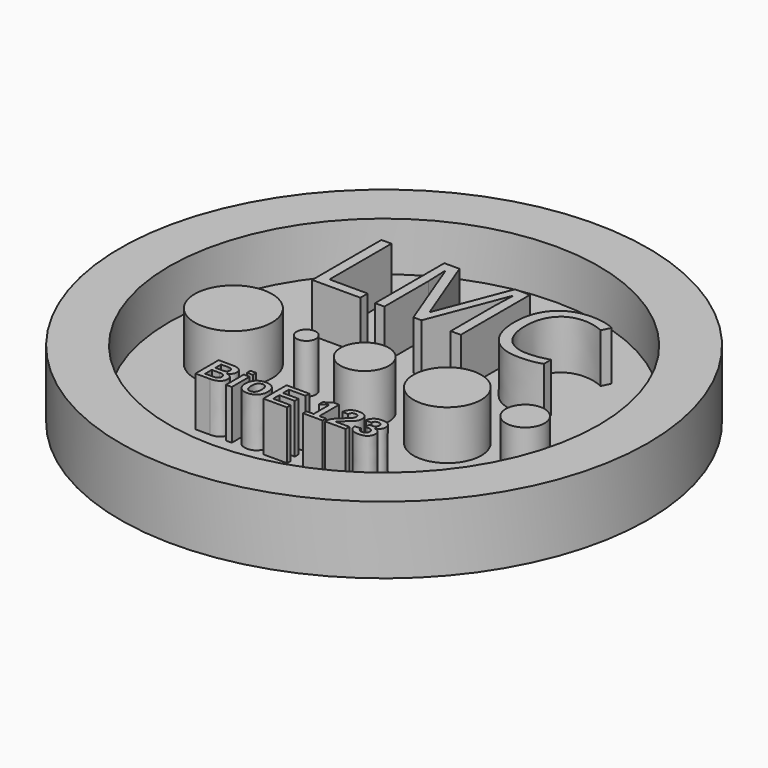
from build123d import *

# Parameters (mm, degrees)
F0_R         = 22.225
F1_DEPTH     = 1.905
F0_R_2       = 27.305
F2_DEPTH     = 6.985
F3_R         = 4.0005
F3_R_2       = 1.0033
F3_R_3       = 2.5019
F3_R_4       = 3.5052
F3_R_5       = 2.0066
F4_DEPTH     = 6.985
F5_TEXT_SIZE = 12.5402686082
F6_DEPTH     = 6.985
F7_TEXT_SIZE = 4.3600920921
F8_DEPTH     = 6.985


# Not quite as in the source:
# - Text() gives the source's letters only with a copy of the font that has no kerning and outlines rounded to 1/6400 em; it was checked with that copy


with BuildPart() as f1:
    # F0 (on Top) → F1 (new body)
    with BuildSketch(Plane.XY):
        Circle(F0_R)
    extrude(amount=F1_DEPTH)

    # F0 (on Top) → F2 (join)
    with BuildSketch(Plane.XY):
        Circle(F0_R_2)
        Circle(F0_R, mode=Mode.SUBTRACT)
    extrude(amount=F2_DEPTH)

    # F3 (on Top) → F4 (join)
    with BuildSketch(Plane.XY):
        with Locations((-13.589, -2.5019)):
            Circle(F3_R)
        with Locations((-6.0452, -2.5019)):
            Circle(F3_R_2)
        with Locations((0, -2.5019)):
            Circle(F3_R_3)
        with Locations((8.5471, -2.5019)):
            Circle(F3_R_4)
        with Locations((16.5989, -2.5019)):
            Circle(F3_R_5)
    extrude(amount=F4_DEPTH)

    # F5 (on Top) → F6 (join)
    with BuildSketch(Plane.XY):
        with Locations((-12.9483295535, 5.3467)):
            Text('LMC', F5_TEXT_SIZE, font='Open Sans', text_align=(TextAlign.LEFT, TextAlign.BOTTOM))
    extrude(amount=F6_DEPTH)

    # F7 (on Top) → F8 (join)
    with BuildSketch(Plane.XY):
        with Locations((-9.1383295535, -13.3342382126)):
            Text('BioE 123', F7_TEXT_SIZE, font='Arimo', font_style=FontStyle.BOLD, text_align=(TextAlign.LEFT, TextAlign.BOTTOM))
    extrude(amount=F8_DEPTH)


solid = f1.part
